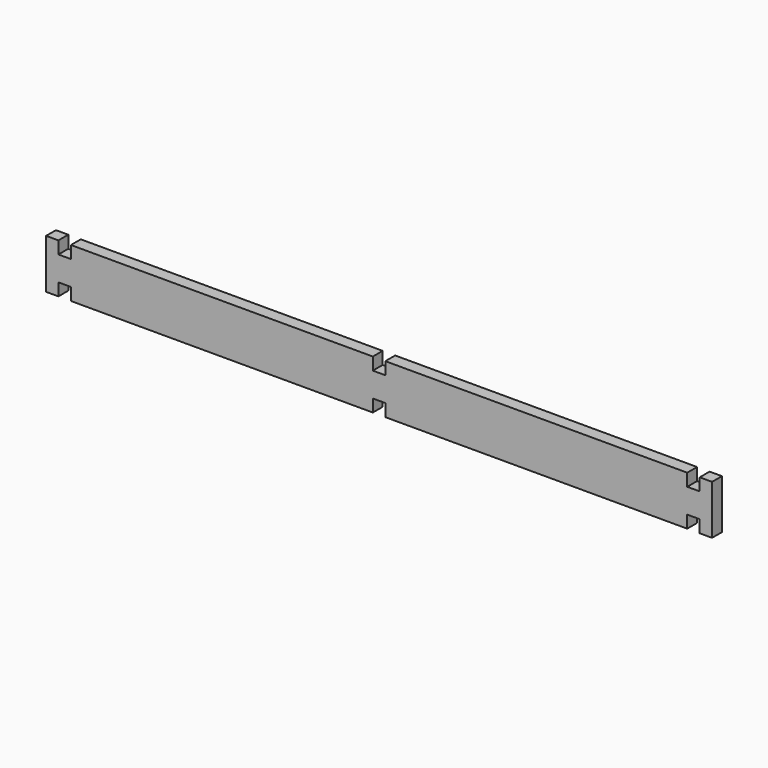
from build123d import *

# Parameters (mm, degrees)
F1_DEPTH = 3


# Not quite as in the source:
# - a feature names something its author has since deleted; it is built from what else it names


with BuildPart() as f1:
    # F0 (on Front) → F1 (new body)
    with BuildSketch(Plane.XZ):
        Polygon((-81.04, 0), (-78.04, 0), (-78.04, 3.02), (-75, 3.02), (-75, 0), (-1.52, 0), (-1.52, 3.02), (1.52, 3.02), (1.52, 0), (75, 0), (75, 3.02), (78.04, 3.02), (78.04, 0), (81.04, 0), (81.04, 12), (78.04, 12), (78.04, 8.98), (75, 8.98), (75, 12), (1.52, 12), (1.52, 8.98), (-1.52, 8.98), (-1.52, 12), (-75, 12), (-75, 8.98), (-78.04, 8.98), (-78.04, 12), (-81.04, 12), align=None)
    extrude(amount=F1_DEPTH)


solid = f1.part
